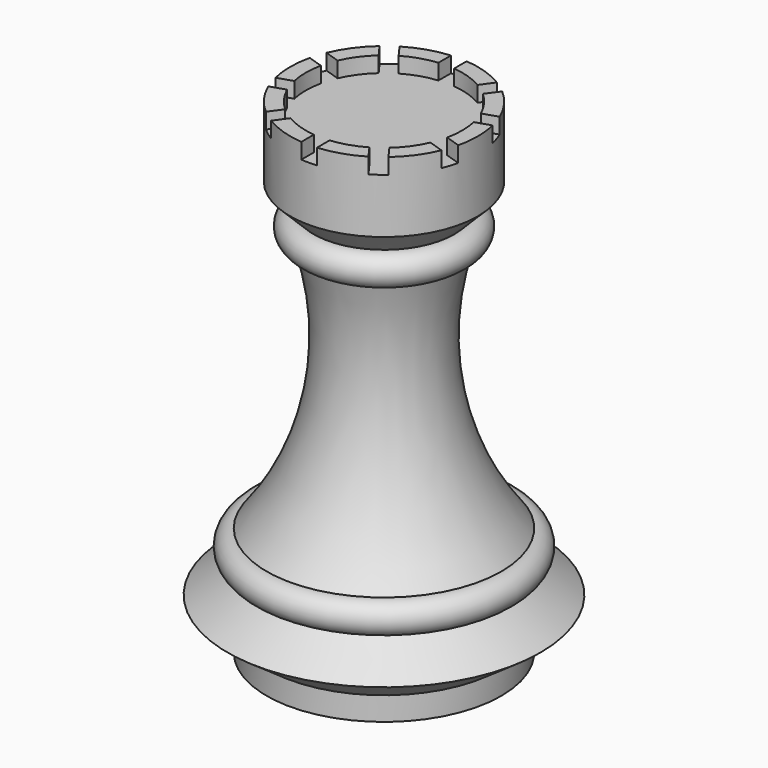
from build123d import *

# Parameters (mm, degrees)
F2_W            = 2.54
F2_H            = 2.54
F3_DEPTH        = 25.4
F3_DEPTH_BACK   = 25.401
F3_COPIES_COUNT = 5
F3_COPIES_ANGLE = 144


# Not quite as in the source:
# - a pattern or mirror of a feature is missing from the dataset's text; its kind, count and spacing are read off the source's solid


with BuildPart() as f1:
    # F0 (on Front) → F1 (revolve)
    with BuildSketch(Plane.XZ):
        with BuildLine():
            Line((0, 76.2), (0, 0))
            Line((0, 0), (19.05, 0))
            Line((19.05, 0), (19.05, 3.81))
            Line((19.05, 3.81), (25.4, 8.255))
            Line((25.4, 8.255), (19.05, 12.7))
            ThreePointArc((19.05, 12.7), (21.59, 15.24), (19.05, 17.78))
            ThreePointArc((19.05, 17.78), (10.2268710231, 37.1600383168), (11.43, 58.42))
            ThreePointArc((11.43, 58.42), (13.97, 60.96), (11.43, 63.5))
            Line((11.43, 63.5), (15.24, 67.31))
            Line((15.24, 67.31), (15.24, 78.74))
            Line((15.24, 78.74), (12.7, 78.74))
            Line((12.7, 78.74), (12.7, 76.2))
            Line((12.7, 76.2), (0, 76.2))
        make_face()
    revolve(axis=Axis((0, 0, 38.1), (0, 0, 1)))

    # F2 (on Front) → F3 (cut, two sides)
    with BuildSketch(Plane.XZ) as f3_sk:
        with Locations((0, 77.47)):
            Rectangle(F2_W, F2_H)
    f3 = extrude(amount=-F3_DEPTH, mode=Mode.SUBTRACT) + extrude(f3_sk.sketch, amount=F3_DEPTH_BACK, mode=Mode.SUBTRACT)

    # F3_copies: F3 ×5 about axis
    f3_copies_axis = Axis((0, 0, 0), (0, 0, 1))
    for i in range(1, F3_COPIES_COUNT):
        add(f3.rotate(f3_copies_axis, i * F3_COPIES_ANGLE / (F3_COPIES_COUNT - 1)), mode=Mode.SUBTRACT)


solid = f1.part
